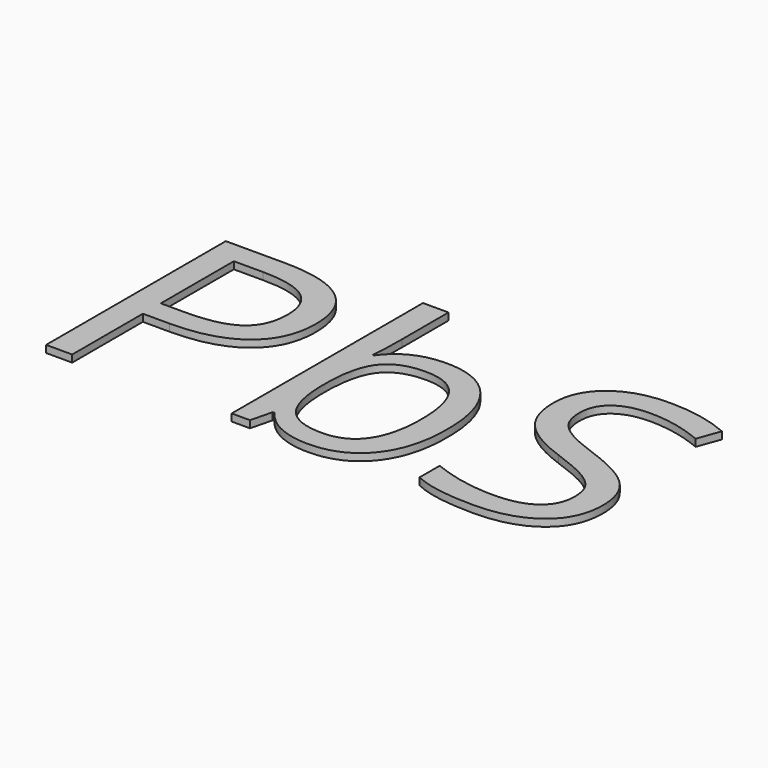
from build123d import *

# Parameters (mm, degrees)
F0_TEXT_SIZE = 43.8514501891
F1_DEPTH     = 1


# Not quite as in the source:
# - Text() gives the source's letters only with a copy of the font that has no kerning and outlines rounded to 1/6400 em; it was checked with that copy


with BuildPart() as f1:
    # F0 (on Top) → F1 (new body)
    with BuildSketch(Plane.XY):
        with Locations((-41.4754939266, -12.772728689)):
            Text('PbS', F0_TEXT_SIZE, font='Open Sans', text_align=(TextAlign.LEFT, TextAlign.BOTTOM))
    extrude(amount=F1_DEPTH)


solid = f1.part
